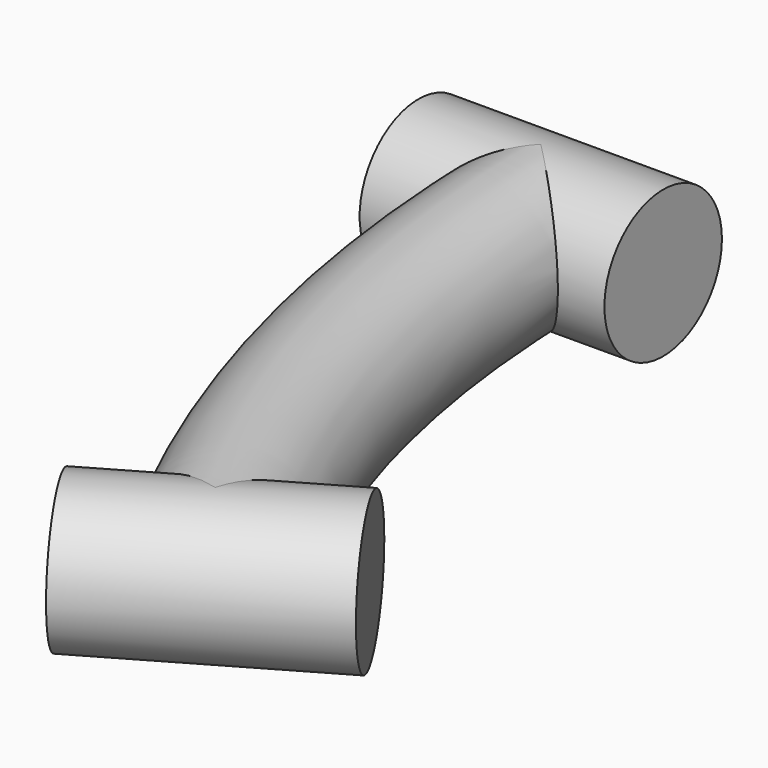
from build123d import *

# Parameters (mm, degrees)
F0_R     = 3.81
F4_R     = 3.81
F5_DEPTH = 6.35
F8_R     = 3.81
F9_DEPTH = 6.35


with BuildPart() as f2:
    # F2: sweep along a path in F1
    with BuildLine(Plane.XY) as f2_path:
        ThreePointArc((0, 0), (2.5964520368, -19.7220112368), (10.2088642316, -38.1))
    # F0 (on Front) → F2 (sweep)
    with BuildSketch(Plane.XZ):
        with Locations((12.7, 0)):
            Circle(F0_R)
    sweep(path=f2_path.line)

    # F4 (on offset) → F5 (join, symmetric)
    with BuildSketch(Plane.YZ.offset(12.7)):
        Circle(F4_R)
    extrude(amount=F5_DEPTH, both=True)

    # F8 (on face) → F9 (join, symmetric)
    with BuildSketch(Plane(origin=(2.1573868597, 1.2455678842, 0), x_dir=(-0.5, 0.8660254038, 0), z_dir=(0.8660254038, 0.5, 0))):
        with Locations((-38.1, 0)):
            Circle(F8_R)
    extrude(amount=F9_DEPTH, both=True)


solid = f2.part
